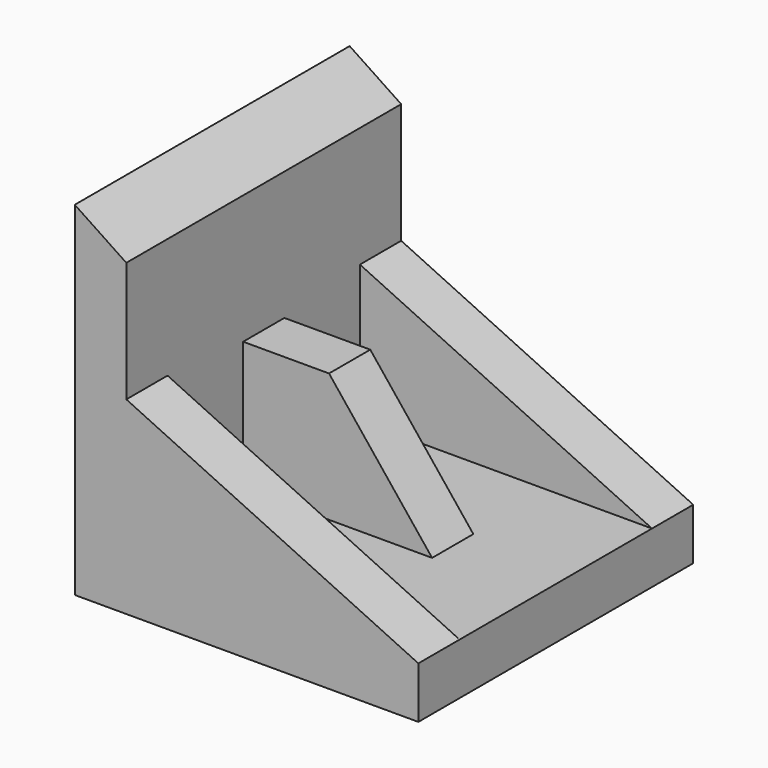
from build123d import *

# Parameters (mm, degrees)
F1_DEPTH = 127
F3_DEPTH = 38.1
F4_DEPTH = 19.05


# Not quite as in the source:
# - a pattern or mirror of a feature is missing from the dataset's text; its kind, count and spacing are read off the source's solid


with BuildPart() as f1:
    # F0 (on Front) → F1 (new body, symmetric)
    with BuildSketch(Plane.XZ):
        Polygon((0, 254), (0, 0), (254, 0), (254, 38.1), (177.8, 38.1), (38.1, 38.1), (38.1, 133.35), (38.1, 228.6), align=None)
    extrude(amount=F1_DEPTH, both=True)

    # F2 (on face) → F3 (join)
    with BuildSketch(Plane.XZ.offset(127)):
        Polygon((254, 38.1), (38.1, 139.7), (38.1, 38.1), align=None)
    f3 = extrude(amount=-F3_DEPTH)

    # F3_copies: F3 across plane
    add(f3.mirror(Plane.ZX))

    # F0 (on Front) → F4 (join, symmetric)
    with BuildSketch(Plane.XZ):
        Polygon((0, 254), (0, 0), (254, 0), (254, 38.1), (177.8, 38.1), (38.1, 38.1), (38.1, 133.35), (38.1, 228.6), align=None)
        Polygon((101.6, 133.35), (38.1, 133.35), (38.1, 38.1), (177.8, 38.1), align=None)
    extrude(amount=F4_DEPTH, both=True)


solid = f1.part
